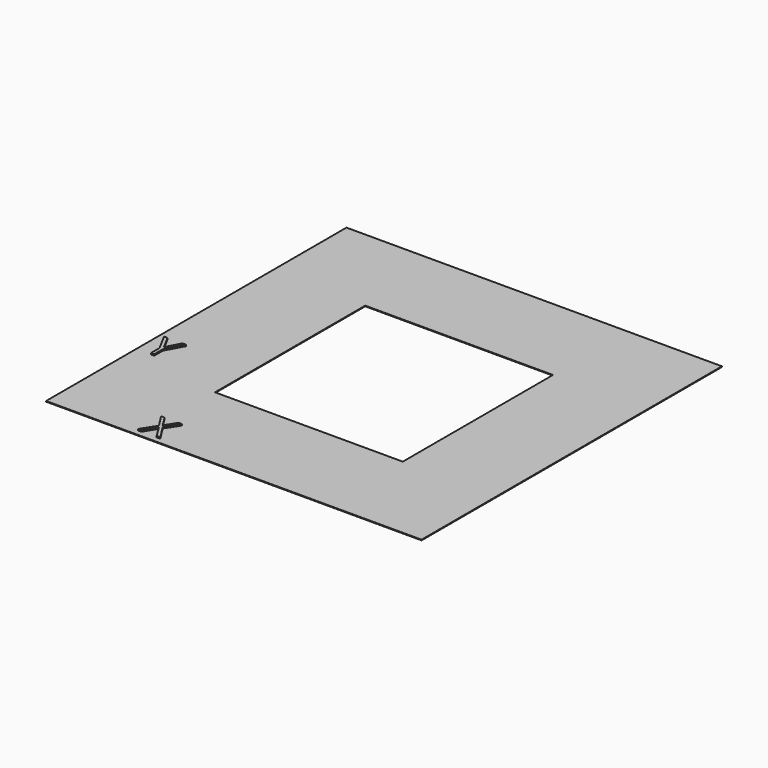
from build123d import *

# Parameters (mm, degrees)
F0_W         = 100
F0_H         = 100
F0_W_2       = 50
F0_H_2       = 50
F1_DEPTH     = 0.175
F2_TEXT_SIZE = 10.4487666653
F3_DEPTH     = 0.35


# Not quite as in the source:
# - Text() gives the source's letters only with a copy of the font that has no kerning and outlines rounded to 1/6400 em; it was checked with that copy


with BuildPart() as f1:
    # F0 (on Top) → F1 (new body)
    with BuildSketch(Plane.XY):
        with Locations((14.28270787, -7.3281310499)):
            Rectangle(F0_W, F0_H)
        with Locations((14.28270787, -7.3281310499)):
            Rectangle(F0_W_2, F0_H_2, mode=Mode.SUBTRACT)
    extrude(amount=F1_DEPTH)

    # F2 (on face) → F3 (join)
    with BuildSketch(Plane.XY.offset(0.175)):
        with Locations((-34.2535031959, -27.3493174464)):
            Text('Y', F2_TEXT_SIZE, font='Open Sans', text_align=(TextAlign.LEFT, TextAlign.BOTTOM))
        with Locations((-12.5331294904, -55.769962776)):
            Text('X', F2_TEXT_SIZE, font='Open Sans', text_align=(TextAlign.LEFT, TextAlign.BOTTOM))
    extrude(amount=F3_DEPTH)


solid = f1.part
